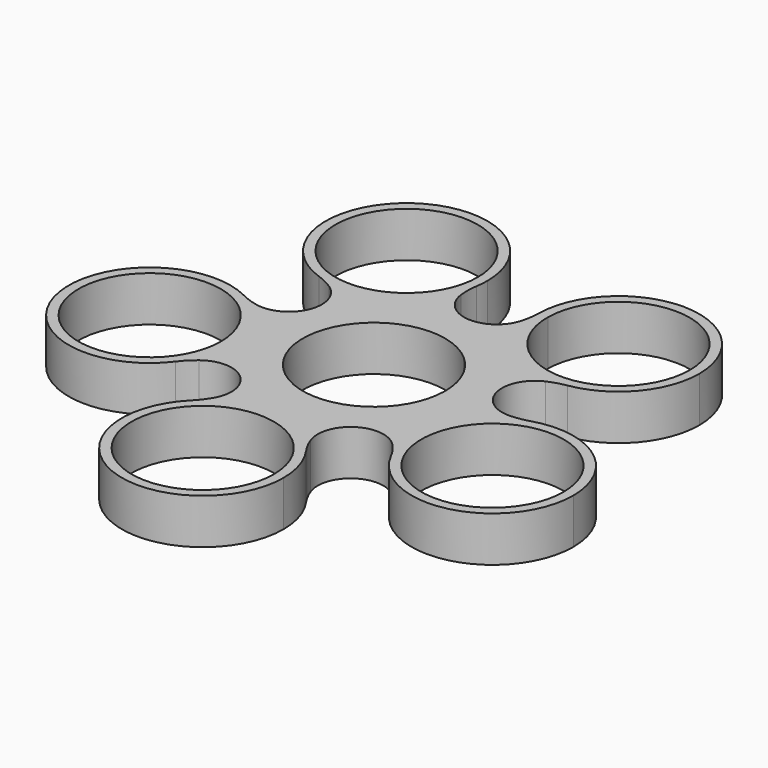
from build123d import *

# Parameters (mm, degrees)
F0_R        = 11
F1_DEPTH    = 7
F2_T1_DEPTH = 7


# Not quite as in the source:
# - a fillet or chamfer that OpenCascade refuses, or shapes differently, is made with other operations: its cross-section is extruded or revolved along the edge and cut away or added


with BuildPart() as f1:
    # F0 (on Top) → F1 (new body)
    with BuildSketch(Plane.XY):
        with BuildLine():
            ThreePointArc((-9.9988986959, 7.5014681809), (-6.4607179934, 10.7008935613), (-1.9816481289, 12.341923298))
            ThreePointArc((-1.9816481289, 12.341923298), (-0.3831736882, 12.7248418239), (1.1389923545, 13.3451302033))
            ThreePointArc((1.1389923545, 13.3451302033), (-2.4661233688, 17.9474854132), (-3.1554936593, 23.7529398707))
            ThreePointArc((-3.1554936593, 23.7529398707), (-9.0450051907, 14.9812509858), (-19.5502137573, 13.8545456359))
            ThreePointArc((-19.5502137573, 13.8545456359), (-14.7338220094, 10.5408010189), (-12.3400050466, 5.2071181257))
            ThreePointArc((-12.3400050466, 5.2071181257), (-11.0821926148, 6.2652556505), (-9.9988986959, 7.5014681809))
        make_face()
        with BuildLine():
            ThreePointArc((8.8575875126, -8.820042146), (11.5166580742, -4.8596899903), (12.4985313373, -0.1916100485))
            Line((12.4985313373, -0.1916100485), (10.9987075768, -0.1686168427))
            ThreePointArc((10.9987075768, -0.1686168427), (-10.0394748812, -4.4954359199), (7.1990009483, 8.3171140034))
            Line((7.1990009483, 8.3171140034), (8.1806828958, 9.451265913))
            ThreePointArc((8.1806828958, 9.451265913), (6.2269941558, 10.838567423), (4.0444905732, 11.8275989112))
            ThreePointArc((4.0444905732, 11.8275989112), (1.0629967692, 12.4547195018), (-1.9816481289, 12.341923298))
            ThreePointArc((-1.9816481289, 12.341923298), (-6.4607179934, 10.7008935613), (-9.9988986959, 7.5014681809))
            ThreePointArc((-9.9988986959, 7.5014681809), (-11.5166580742, 4.8596899903), (-12.3502295249, 1.9292046764))
            ThreePointArc((-12.3502295249, 1.9292046764), (-12.1736262075, -2.8377499821), (-10.2241498173, -7.1914366098))
            ThreePointArc((-10.2241498173, -7.1914366098), (-8.1806828958, -9.451265913), (-5.6512134863, -11.1496092367))
            ThreePointArc((-5.6512134863, -11.1496092367), (-1.0629967692, -12.4547195018), (3.6800266027, -11.9460204337))
            ThreePointArc((3.6800266027, -11.9460204337), (6.4607179934, -10.7008935613), (8.8575875126, -8.820042146))
        make_face()
        with BuildLine():
            ThreePointArc((-1.9816481289, 12.341923298), (1.0629967692, 12.4547195018), (4.0444905732, 11.8275989112))
            ThreePointArc((4.0444905732, 11.8275989112), (2.5340263598, 12.4758619713), (1.1389923545, 13.3451302033))
            ThreePointArc((1.1389923545, 13.3451302033), (-0.3831736882, 12.7248418239), (-1.9816481289, 12.341923298))
        make_face()
        with BuildLine():
            ThreePointArc((11.1255036275, 5.6985234083), (12.1515183278, 2.930972932), (12.5, 0))
            ThreePointArc((12.5, 0), (12.4996328289, -0.0958078385), (12.4985313373, -0.1916100485))
            ThreePointArc((12.4985313373, -0.1916100485), (12.6483070335, 1.4452510866), (13.0439410346, 3.0406259242))
            ThreePointArc((13.0439410346, 3.0406259242), (11.983636554, 4.2966122073), (11.1255036275, 5.6985234083))
        make_face()
        with BuildLine():
            ThreePointArc((12.4985313373, -0.1916100485), (12.4996328289, -0.0958078385), (12.5, 0))
            ThreePointArc((12.5, 0), (12.1515183278, 2.930972932), (11.1255036275, 5.6985234083))
            ThreePointArc((11.1255036275, 5.6985234083), (9.8337672636, 7.7166716533), (8.1806828958, 9.451265913))
            Line((8.1806828958, 9.451265913), (7.1990009483, 8.3171140034))
            ThreePointArc((7.1990009483, 8.3171140034), (10.0047241449, 4.5722527035), (11, 0))
            ThreePointArc((11, 0), (10.9996768895, -0.0843108979), (10.9987075768, -0.1686168427))
            Line((10.9987075768, -0.1686168427), (12.4985313373, -0.1916100485))
        make_face()
        with BuildLine():
            ThreePointArc((-12.3502295249, 1.9292046764), (-11.5166580742, 4.8596899903), (-9.9988986959, 7.5014681809))
            ThreePointArc((-9.9988986959, 7.5014681809), (-11.0821926148, 6.2652556505), (-12.3400050466, 5.2071181257))
            ThreePointArc((-12.3400050466, 5.2071181257), (-12.2204509169, 3.5677725413), (-12.3502295249, 1.9292046764))
        make_face()
        with BuildLine():
            ThreePointArc((-8.7655348947, -10.1269542181), (-9.3831980656, -8.603721031), (-10.2241498173, -7.1914366098))
            ThreePointArc((-10.2241498173, -7.1914366098), (-12.1736262075, -2.8377499821), (-12.3502295249, 1.9292046764))
            ThreePointArc((-12.3502295249, 1.9292046764), (-12.2204509169, 3.5677725413), (-12.3400050466, 5.2071181257))
            ThreePointArc((-12.3400050466, 5.2071181257), (-17.8311469845, 3.2006552991), (-23.5654894116, 4.3390092796))
            ThreePointArc((-23.5654894116, 4.3390092796), (-18.5656426554, -0.2680533802), (-16.7167028979, -6.8105999571))
            ThreePointArc((-16.7167028979, -6.8105999571), (-17.3584518949, -10.7643175938), (-19.217804202, -14.312068138))
            ThreePointArc((-19.217804202, -14.312068138), (-14.577898889, -10.7554107829), (-8.7655348947, -10.1269542181))
        make_face()
        with BuildLine():
            ThreePointArc((8.1806828958, 9.451265913), (9.8337672636, 7.7166716533), (11.1255036275, 5.6985234083))
            ThreePointArc((11.1255036275, 5.6985234083), (11.983636554, 4.2966122073), (13.0439410346, 3.0406259242))
            ThreePointArc((13.0439410346, 3.0406259242), (16.3069989221, 7.8915006988), (21.6152870788, 10.3411148932))
            ThreePointArc((21.6152870788, 10.3411148932), (16.2136999096, 10.6599763116), (11.4529560542, 13.2317722782))
            Line((11.4529560542, 13.2317722782), (8.1806828958, 9.451265913))
        make_face()
        with BuildLine():
            ThreePointArc((13.0439410346, 3.0406259242), (12.6483070335, 1.4452510866), (12.4985313373, -0.1916100485))
            ThreePointArc((12.4985313373, -0.1916100485), (11.5166580742, -4.8596899903), (8.8575875126, -8.820042146))
            ThreePointArc((8.8575875126, -8.820042146), (7.7894683874, -10.0693894433), (6.9226065521, -11.4659200351))
            ThreePointArc((6.9226065521, -11.4659200351), (12.5444029571, -13.0702697591), (16.5144757506, -17.3617793852))
            ThreePointArc((16.5144757506, -17.3617793852), (16.1233213039, -6.8035659865), (23.9599527753, 0.2827644569))
            ThreePointArc((23.9599527754, 0.2827644569), (18.115639784, 0.1326361285), (13.0439410346, 3.0406259242))
        make_face()
        with BuildLine():
            ThreePointArc((4.0444905732, 11.8275989112), (6.2269941558, 10.838567423), (8.1806828958, 9.451265913))
            Line((8.1806828958, 9.451265913), (11.4529560542, 13.2317722782))
            ThreePointArc((11.4529560542, 13.2317722782), (8.2251447668, 17.5745882822), (7.1351076127, 22.8746482397))
            ThreePointArc((7.1351076127, 22.8746482397), (5.471896103, 17.2699840812), (1.1389923545, 13.3451302033))
            ThreePointArc((1.1389923545, 13.3451302033), (2.5340263598, 12.4758619713), (4.0444905732, 11.8275989112))
        make_face()
        with BuildLine():
            ThreePointArc((6.9226065521, -11.4659200351), (7.7894683874, -10.0693894433), (8.8575875126, -8.820042146))
            ThreePointArc((8.8575875126, -8.820042146), (6.4607179934, -10.7008935613), (3.6800266027, -11.9460204337))
            ThreePointArc((3.6800266027, -11.9460204337), (5.2830572871, -11.5826476774), (6.9226065521, -11.4659200351))
        make_face()
        with BuildLine():
            ThreePointArc((-8.7655348947, -10.1269542181), (-7.1694803363, -10.5198371292), (-5.6512134863, -11.1496092367))
            ThreePointArc((-5.6512134863, -11.1496092367), (-8.1806828958, -9.451265913), (-10.2241498173, -7.1914366098))
            ThreePointArc((-10.2241498173, -7.1914366098), (-9.3831980656, -8.603721031), (-8.7655348947, -10.1269542181))
        make_face()
        with BuildLine():
            ThreePointArc((6.9226065521, -11.4659200351), (5.2830572871, -11.5826476774), (3.6800266027, -11.9460204337))
            ThreePointArc((3.6800266027, -11.9460204337), (-1.0629967692, -12.4547195018), (-5.6512134863, -11.1496092367))
            ThreePointArc((-5.6512134863, -11.1496092367), (-7.1694803363, -10.5198371292), (-8.7655348947, -10.1269542181))
            ThreePointArc((-8.7655348947, -10.1269542181), (-8.554131526, -15.969371652), (-11.4087797586, -21.0712846584))
            ThreePointArc((-11.4087797586, -21.0712846584), (-1.4881954768, -17.4366073025), (7.6729575713, -22.6998901945))
            ThreePointArc((7.6729575713, -22.6998901945), (5.7241850115, -17.1880104456), (6.9226065521, -11.4659200351))
        make_face()
        with BuildLine():
            ThreePointArc((40.139979378, -11.6632559768), (35.0645893835, -1.6071550293), (23.9599527753, 0.2827644569))
            ThreePointArc((23.9599527753, 0.2827644569), (16.1233213039, -6.8035659865), (16.5144757506, -17.3617793852))
            ThreePointArc((16.5144757506, -17.3617793852), (30.5709523101, -23.8147743047), (40.139979378, -11.6632559768))
        make_face()
        with Locations((27.639979378, -11.6632559768)):
            Circle(F0_R, mode=Mode.SUBTRACT)
        with BuildLine():
            ThreePointArc((9.948807754, -29.8913268043), (9.3662712575, -26.1198465059), (7.6729575713, -22.6998901945))
            ThreePointArc((7.6729575713, -22.6998901945), (-1.4881954768, -17.4366073025), (-11.4087797586, -21.0712846584))
            ThreePointArc((-11.4087797586, -21.0712846584), (-7.3224686, -41.4448943033), (9.948807754, -29.8913268043))
        make_face()
        with Locations((-2.551192246, -29.8913268043)):
            Circle(F0_R, mode=Mode.SUBTRACT)
        with BuildLine():
            ThreePointArc((-23.5654894116, 4.3390092796), (-41.3903291054, -9.6483499392), (-19.217804202, -14.312068138))
            ThreePointArc((-19.217804202, -14.312068138), (-17.3584518949, -10.7643175938), (-16.7167028979, -6.8105999571))
            ThreePointArc((-16.7167028979, -6.8105999571), (-18.5656426554, -0.2680533802), (-23.5654894116, 4.3390092796))
        make_face()
        with Locations((-29.2167028979, -6.8105999571)):
            Circle(F0_R, mode=Mode.SUBTRACT)
        with BuildLine():
            ThreePointArc((-19.5502137573, 13.8545456359), (-9.0450051907, 14.9812509858), (-3.1554936593, 23.7529398707))
            ThreePointArc((-3.1554936593, 23.7529398707), (-3.0432220495, 24.7146397824), (-3.0057231841, 25.6821445471))
            ThreePointArc((-3.0057231841, 25.6821445471), (-22.7753128505, 35.8508743637), (-19.5502137573, 13.8545456359))
        make_face()
        with Locations((-15.5057231841, 25.6821445471)):
            Circle(F0_R, mode=Mode.SUBTRACT)
        with BuildLine():
            Line((21.3774893034, 11.8221456889), (21.6152870788, 10.3411148932))
            ThreePointArc((21.6152870788, 10.3411148932), (29.1473291281, 14.5750360208), (32.13363895, 22.6830381912))
            ThreePointArc((32.13363895, 22.6830381912), (19.7294467885, 35.1826710201), (7.1351076127, 22.8746482397))
            Line((7.1351076127, 22.8746482397), (8.6349313732, 22.8516550339))
            ThreePointArc((8.6349313732, 22.8516550339), (19.7179498479, 33.6827150806), (30.63363895, 22.6830381912))
            ThreePointArc((30.63363895, 22.6830381912), (28.0056863067, 15.5479962813), (21.3774893034, 11.8221456889))
        make_face()
        with BuildLine():
            ThreePointArc((7.1351076127, 22.8746482397), (8.2251447668, 17.5745882822), (11.4529560542, 13.2317722782))
            Line((11.4529560542, 13.2317722782), (12.4346380016, 14.3659241877))
            ThreePointArc((12.4346380016, 14.3659241877), (9.5941640688, 18.1876022712), (8.6349313732, 22.8516550339))
            Line((8.6349313732, 22.8516550339), (7.1351076127, 22.8746482397))
        make_face()
        with BuildLine():
            Line((12.4346380016, 14.3659241877), (11.4529560542, 13.2317722782))
            ThreePointArc((11.4529560542, 13.2317722782), (16.2136999096, 10.6599763116), (21.6152870788, 10.3411148932))
            Line((21.6152870788, 10.3411148932), (21.3774893034, 11.8221456889))
            ThreePointArc((21.3774893034, 11.8221456889), (16.6240925945, 12.1027437371), (12.4346380016, 14.3659241877))
        make_face()
    extrude(amount=F1_DEPTH)

    # F2: fillet of radius 5.08 on 5 edges, made by hand

    # F2_s2 → F2_t1 (join)
    with BuildSketch(Plane.XY):
        with BuildLine():
            ThreePointArc((6.3459415764, -20.1508962512), (8.4975237439, -14.0744569275), (14.876798383, -15.0003487989))
            ThreePointArc((14.876798383, -15.0003487989), (11.2701865952, -12.3993640914), (6.9226065521, -11.4659200351))
            ThreePointArc((6.9226065521, -11.4659200351), (5.7239018226, -15.7479612549), (6.3459415764, -20.1508962512))
        make_face()
        with BuildLine():
            ThreePointArc((-17.2036373964, -12.2623184818), (-10.7597247272, -12.4308717062), (-9.6689959497, -18.7840387442))
            ThreePointArc((-9.6689959497, -18.7840387442), (-8.3098168293, -14.5501986249), (-8.7655348947, -10.1269542181))
            ThreePointArc((-8.7655348947, -10.1269542181), (-13.2084182325, -10.3101417816), (-17.2036373964, -12.2623184818))
        make_face()
        with BuildLine():
            ThreePointArc((-16.9783742176, 12.5723666486), (-15.147399335, 6.3917557032), (-20.852566517, 3.391174409))
            ThreePointArc((-20.852566517, 3.391174409), (-16.405935836, 3.4068467981), (-12.3400050466, 5.2071181257))
            ThreePointArc((-12.3400050466, 5.2071181257), (-13.8871532279, 9.3759432051), (-16.9783742176, 12.5723666486))
        make_face()
        with BuildLine():
            ThreePointArc((6.7104250563, 20.0324683896), (1.398117097, 16.3811939786), (-3.2185989105, 20.8798997907))
            ThreePointArc((-3.2185989105, 20.8798997907), (-1.8296091346, 16.6557457406), (1.1389923545, 13.3451302033))
            ThreePointArc((1.1389923545, 13.3451302033), (4.6256855307, 16.1047933589), (6.7104250563, 20.0324683896))
        make_face()
        with BuildLine():
            ThreePointArc((18.8633629941, 9.5133133434), (16.0114832212, 3.7323789519), (21.1256449813, -0.1916203052))
            ThreePointArc((21.1256449813, -0.1916203052), (16.7459841072, 0.5773664725), (13.0439410346, 3.0406259242))
            ThreePointArc((13.0439410346, 3.0406259242), (15.2751752047, 6.8869701775), (18.8633629941, 9.5133133434))
        make_face()
    extrude(amount=F2_T1_DEPTH)


solid = f1.part
